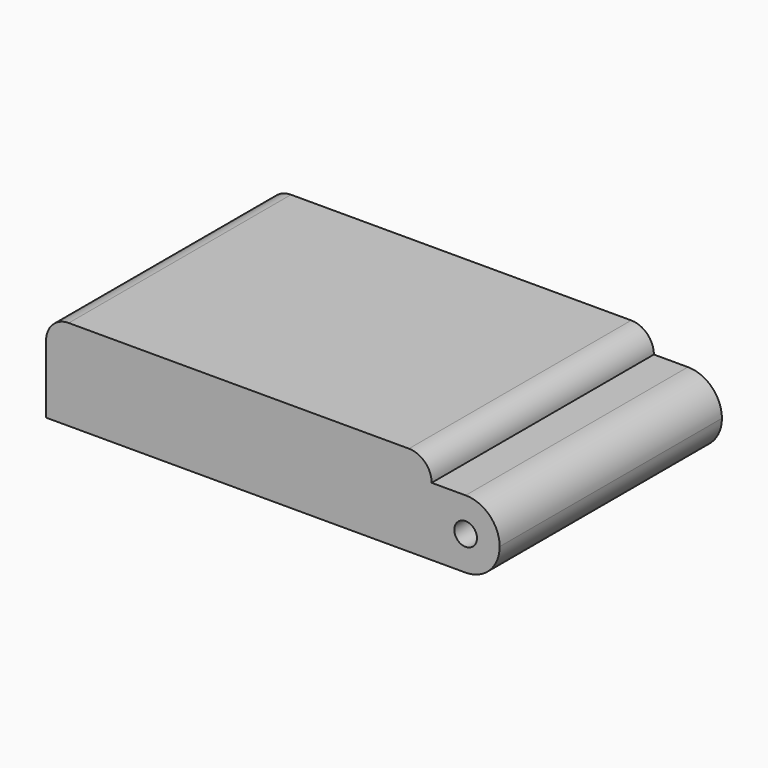
from build123d import *

# Parameters (mm, degrees)
F0_W     = 40
F0_H     = 24.5
F1_DEPTH = 8
F2_T     = -2
F3_R     = 1
F4_DEPTH = 25
F5_R     = 1.99999
F7_DEPTH = 22.5


# Not quite as in the source:
# - a fillet or chamfer is up to 0.001 mm smaller than in the source, because OpenCascade refuses the exact size


with BuildPart() as f1:
    # F0 (on Top) → F1 (new body)
    with BuildSketch(Plane.XY):
        Rectangle(F0_W, F0_H)
    extrude(amount=F1_DEPTH)

    # F2
    f2_openings = [f1.faces().sort_by_distance(p)[0] for p in [
        (0, 0, 0),
    ]]
    offset(amount=F2_T, openings=f2_openings)

    # F3 (on face) → F4 (cut)
    with BuildSketch(Plane.XZ.offset(12.25)):
        with Locations((17, 3)):
            Circle(F3_R)
        with BuildLine():
            ThreePointArc((17, 6), (19.1213203436, 5.1213203436), (20, 3))
            Line((20, 3), (20, 8))
            Line((20, 8), (14, 8))
            Line((14, 8), (14, 6))
            Line((14, 6), (17, 6))
        make_face()
        with BuildLine():
            ThreePointArc((20, 3), (19.1213203436, 0.8786796564), (17, 0))
            Line((17, 0), (20, 0))
            Line((20, 0), (20, 3))
        make_face()
    extrude(amount=-F4_DEPTH, mode=Mode.SUBTRACT)

    # F5 (radius 2 in the source; OpenCascade refuses exactly that, so slightly less here)
    f5_edges = [f1.edges().sort_by_distance(p)[0] for p in [
        (-20, 0, 8),
        (14, 0, 8),
    ]]
    fillet(f5_edges, radius=F5_R)

    # F6 (on face) → F7 (join)
    with BuildSketch(Plane.XZ.offset(-10.25)):
        with BuildLine():
            Line((14, 6), (13.095, 6))
            Line((13.095, 6), (13.095, 4.4142135624))
            Line((13.095, 4.4142135624), (18, 4.4142135624))
            Line((18, 4.4142135624), (18, 5.8284271247))
            ThreePointArc((18, 5.8284271247), (17.5073059362, 5.956795679), (17, 6))
            Line((17, 6), (14, 6))
        make_face()
    extrude(amount=F7_DEPTH)


solid = f1.part
